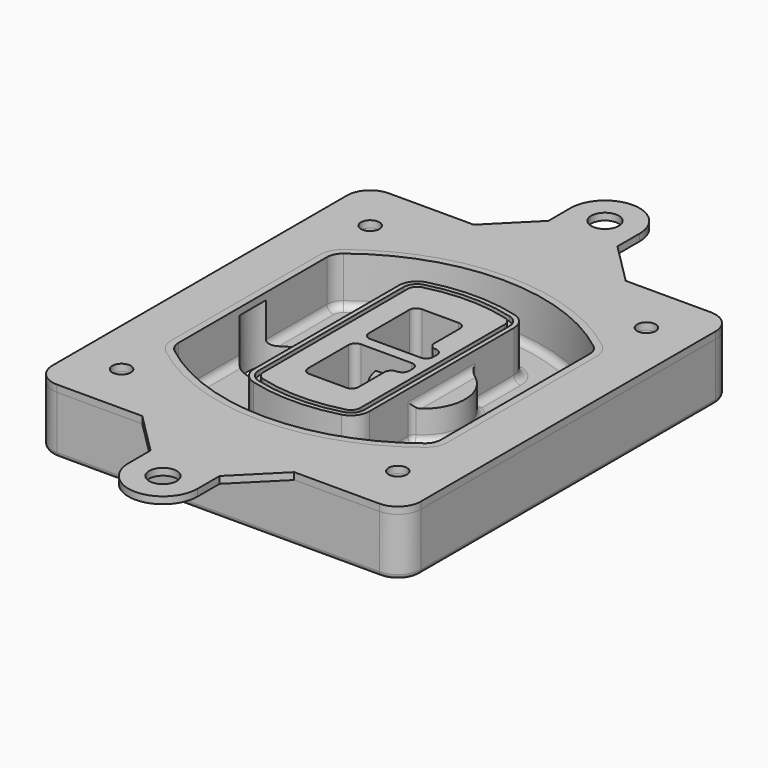
from build123d import *

# Parameters (mm, degrees)
F0_R      = 4
F1_DEPTH  = 25
F2_DEPTH  = 3
F3_DEPTH  = 18
F5_DEPTH  = 21
F6_DEPTH  = 2
F8_DEPTH  = 20
F9_DEPTH  = 16
F10_DEPTH = 25
F7_R      = 6
F7_R_2    = 4
F11_DEPTH = 6
F13_DEPTH = 9
F14_R     = 3
F15_R     = 2
F16_R     = 6
F16_R_2   = 4
F17_DEPTH = 3


with BuildPart() as f1:
    # F0 (on Top) → F1 (new body)
    with BuildSketch(Plane.XY):
        with BuildLine():
            ThreePointArc((-80, -80), (-77.0710678119, -87.0710678119), (-70, -90))
            Line((-70, -90), (70, -90))
            ThreePointArc((70, -90), (77.0710678119, -87.0710678119), (80, -80))
            Line((80, -80), (80, 80))
            ThreePointArc((80, 80), (77.0710678119, 87.0710678119), (70, 90))
            Line((70, 90), (-70, 90))
            ThreePointArc((-70, 90), (-77.0710678119, 87.0710678119), (-80, 80))
            Line((-80, 80), (-80, -80))
        make_face()
        with Locations((-60, -67.5)):
            Circle(F0_R, mode=Mode.SUBTRACT)
        with Locations((60, -67.5)):
            Circle(F0_R, mode=Mode.SUBTRACT)
        with Locations((-60, 67.5)):
            Circle(F0_R, mode=Mode.SUBTRACT)
        with BuildLine():
            ThreePointArc((-64, 40.2934422872), (-62.5820384798, 46.4328484224), (-58.6153846154, 51.3286200352))
            ThreePointArc((-58.6153846154, 51.3286200352), (0, 71.5), (58.6153846154, 51.3286200352))
            ThreePointArc((58.6153846154, 51.3286200352), (62.5820384798, 46.4328484224), (64, 40.2934422872))
            Line((64, 40.2934422872), (64, -40.2934422872))
            ThreePointArc((64, -40.2934422872), (62.5820384798, -46.4328484224), (58.6153846154, -51.3286200352))
            ThreePointArc((58.6153846154, -51.3286200352), (0, -71.5), (-58.6153846154, -51.3286200352))
            ThreePointArc((-58.6153846154, -51.3286200352), (-62.5820384798, -46.4328484224), (-64, -40.2934422872))
            Line((-64, -40.2934422872), (-64, 40.2934422872))
        make_face(mode=Mode.SUBTRACT)
        with Locations((60, 67.5)):
            Circle(F0_R, mode=Mode.SUBTRACT)
        with BuildLine():
            ThreePointArc((58.6153846154, 51.3286200352), (0, 71.5), (-58.6153846154, 51.3286200352))
            ThreePointArc((-58.6153846154, 51.3286200352), (-62.5820384798, 46.4328484224), (-64, 40.2934422872))
            Line((-64, 40.2934422872), (-64, -40.2934422872))
            ThreePointArc((-64, -40.2934422872), (-62.5820384798, -46.4328484224), (-58.6153846154, -51.3286200352))
            ThreePointArc((-58.6153846154, -51.3286200352), (0, -71.5), (58.6153846154, -51.3286200352))
            ThreePointArc((58.6153846154, -51.3286200352), (62.5820384798, -46.4328484224), (64, -40.2934422872))
            Line((64, -40.2934422872), (64, 40.2934422872))
            ThreePointArc((64, 40.2934422872), (62.5820384798, 46.4328484224), (58.6153846154, 51.3286200352))
        make_face()
        with BuildLine():
            Line((-60, -40.2934422872), (-60, 40.2934422872))
            ThreePointArc((-60, 40.2934422872), (-58.9871703427, 44.6787323838), (-56.1538461538, 48.1757121072))
            ThreePointArc((-56.1538461538, 48.1757121072), (0, 67.5), (56.1538461538, 48.1757121072))
            ThreePointArc((56.1538461538, 48.1757121072), (58.9871703427, 44.6787323838), (60, 40.2934422872))
            Line((60, 40.2934422872), (60, -40.2934422872))
            ThreePointArc((60, -40.2934422872), (58.9871703427, -44.6787323838), (56.1538461538, -48.1757121072))
            ThreePointArc((56.1538461538, -48.1757121072), (0, -67.5), (-56.1538461538, -48.1757121072))
            ThreePointArc((-56.1538461538, -48.1757121072), (-58.9871703427, -44.6787323838), (-60, -40.2934422872))
        make_face(mode=Mode.SUBTRACT)
        with BuildLine():
            ThreePointArc((-56.1538461538, 48.1757121072), (-58.9871703427, 44.6787323838), (-60, 40.2934422872))
            Line((-60, 40.2934422872), (-60, -40.2934422872))
            ThreePointArc((-60, -40.2934422872), (-58.9871703427, -44.6787323838), (-56.1538461538, -48.1757121072))
            ThreePointArc((-56.1538461538, -48.1757121072), (0, -67.5), (56.1538461538, -48.1757121072))
            ThreePointArc((56.1538461538, -48.1757121072), (58.9871703427, -44.6787323838), (60, -40.2934422872))
            Line((60, -40.2934422872), (60, 40.2934422872))
            ThreePointArc((60, 40.2934422872), (58.9871703427, 44.6787323838), (56.1538461538, 48.1757121072))
            ThreePointArc((56.1538461538, 48.1757121072), (0, 67.5), (-56.1538461538, 48.1757121072))
        make_face()
        with BuildLine():
            ThreePointArc((54.3076923077, 45.8110311612), (56.2910192399, 43.3631453548), (57, 40.2934422872))
            Line((57, 40.2934422872), (57, -40.2934422872))
            ThreePointArc((57, -40.2934422872), (56.2910192399, -43.3631453548), (54.3076923077, -45.8110311612))
            ThreePointArc((54.3076923077, -45.8110311612), (0, -64.5), (-54.3076923077, -45.8110311612))
            ThreePointArc((-54.3076923077, -45.8110311612), (-56.2910192399, -43.3631453548), (-57, -40.2934422872))
            Line((-57, -40.2934422872), (-57, 40.2934422872))
            ThreePointArc((-57, 40.2934422872), (-56.2910192399, 43.3631453548), (-54.3076923077, 45.8110311612))
            ThreePointArc((-54.3076923077, 45.8110311612), (0, 64.5), (54.3076923077, 45.8110311612))
        make_face(mode=Mode.SUBTRACT)
        with BuildLine():
            Line((57, -40.2934422872), (57, 40.2934422872))
            ThreePointArc((57, 40.2934422872), (56.2910192399, 43.3631453548), (54.3076923077, 45.8110311612))
            ThreePointArc((54.3076923077, 45.8110311612), (0, 64.5), (-54.3076923077, 45.8110311612))
            ThreePointArc((-54.3076923077, 45.8110311612), (-56.2910192399, 43.3631453548), (-57, 40.2934422872))
            Line((-57, 40.2934422872), (-57, -40.2934422872))
            ThreePointArc((-57, -40.2934422872), (-56.2910192399, -43.3631453548), (-54.3076923077, -45.8110311612))
            ThreePointArc((-54.3076923077, -45.8110311612), (0, -64.5), (54.3076923077, -45.8110311612))
            ThreePointArc((54.3076923077, -45.8110311612), (56.2910192399, -43.3631453548), (57, -40.2934422872))
        make_face()
    extrude(amount=-F1_DEPTH)

    # F0 (on Top) → F2 (join)
    with BuildSketch(Plane.XY):
        with BuildLine():
            ThreePointArc((-56.1538461538, 48.1757121072), (-58.9871703427, 44.6787323838), (-60, 40.2934422872))
            Line((-60, 40.2934422872), (-60, -40.2934422872))
            ThreePointArc((-60, -40.2934422872), (-58.9871703427, -44.6787323838), (-56.1538461538, -48.1757121072))
            ThreePointArc((-56.1538461538, -48.1757121072), (0, -67.5), (56.1538461538, -48.1757121072))
            ThreePointArc((56.1538461538, -48.1757121072), (58.9871703427, -44.6787323838), (60, -40.2934422872))
            Line((60, -40.2934422872), (60, 40.2934422872))
            ThreePointArc((60, 40.2934422872), (58.9871703427, 44.6787323838), (56.1538461538, 48.1757121072))
            ThreePointArc((56.1538461538, 48.1757121072), (0, 67.5), (-56.1538461538, 48.1757121072))
        make_face()
        with BuildLine():
            ThreePointArc((54.3076923077, 45.8110311612), (56.2910192399, 43.3631453548), (57, 40.2934422872))
            Line((57, 40.2934422872), (57, -40.2934422872))
            ThreePointArc((57, -40.2934422872), (56.2910192399, -43.3631453548), (54.3076923077, -45.8110311612))
            ThreePointArc((54.3076923077, -45.8110311612), (0, -64.5), (-54.3076923077, -45.8110311612))
            ThreePointArc((-54.3076923077, -45.8110311612), (-56.2910192399, -43.3631453548), (-57, -40.2934422872))
            Line((-57, -40.2934422872), (-57, 40.2934422872))
            ThreePointArc((-57, 40.2934422872), (-56.2910192399, 43.3631453548), (-54.3076923077, 45.8110311612))
            ThreePointArc((-54.3076923077, 45.8110311612), (0, 64.5), (54.3076923077, 45.8110311612))
        make_face(mode=Mode.SUBTRACT)
    extrude(amount=F2_DEPTH)

    # F0 (on Top) → F3 (cut)
    with BuildSketch(Plane.XY):
        with BuildLine():
            Line((57, -40.2934422872), (57, 40.2934422872))
            ThreePointArc((57, 40.2934422872), (56.2910192399, 43.3631453548), (54.3076923077, 45.8110311612))
            ThreePointArc((54.3076923077, 45.8110311612), (0, 64.5), (-54.3076923077, 45.8110311612))
            ThreePointArc((-54.3076923077, 45.8110311612), (-56.2910192399, 43.3631453548), (-57, 40.2934422872))
            Line((-57, 40.2934422872), (-57, -40.2934422872))
            ThreePointArc((-57, -40.2934422872), (-56.2910192399, -43.3631453548), (-54.3076923077, -45.8110311612))
            ThreePointArc((-54.3076923077, -45.8110311612), (0, -64.5), (54.3076923077, -45.8110311612))
            ThreePointArc((54.3076923077, -45.8110311612), (56.2910192399, -43.3631453548), (57, -40.2934422872))
        make_face()
    extrude(amount=-F3_DEPTH, mode=Mode.SUBTRACT)

    # F4 (on face) → F5 (join, through all)
    with BuildSketch(Plane.XY.offset(3)):
        with BuildLine():
            ThreePointArc((-25, -39.2465276821), (-23.3511545998, -44.1109737193), (-19.0842911877, -46.9702398883))
            ThreePointArc((-19.0842911877, -46.9702398883), (0, -49.5), (19.0842911877, -46.9702398883))
            ThreePointArc((19.0842911877, -46.9702398883), (23.3511545998, -44.1109737193), (25, -39.2465276821))
            Line((25, -39.2465276821), (25, 39.2465276821))
            ThreePointArc((25, 39.2465276821), (23.3511545998, 44.1109737193), (19.0842911877, 46.9702398883))
            ThreePointArc((19.0842911877, 46.9702398883), (0, 49.5), (-19.0842911877, 46.9702398883))
            ThreePointArc((-19.0842911877, 46.9702398883), (-23.3511545998, 44.1109737193), (-25, 39.2465276821))
            Line((-25, 39.2465276821), (-25, -39.2465276821))
        make_face()
        with BuildLine():
            ThreePointArc((18.5632183908, 45.0393118368), (21.7633659499, 42.89486221), (23, 39.2465276821))
            Line((23, 39.2465276821), (23, -39.2465276821))
            ThreePointArc((23, -39.2465276821), (21.7633659499, -42.89486221), (18.5632183908, -45.0393118368))
            ThreePointArc((18.5632183908, -45.0393118368), (0, -47.5), (-18.5632183908, -45.0393118368))
            ThreePointArc((-18.5632183908, -45.0393118368), (-21.7633659499, -42.89486221), (-23, -39.2465276821))
            Line((-23, -39.2465276821), (-23, 39.2465276821))
            ThreePointArc((-23, 39.2465276821), (-21.7633659499, 42.89486221), (-18.5632183908, 45.0393118368))
            ThreePointArc((-18.5632183908, 45.0393118368), (0, 47.5), (18.5632183908, 45.0393118368))
        make_face(mode=Mode.SUBTRACT)
        with BuildLine():
            Line((23, -39.2465276821), (23, 39.2465276821))
            ThreePointArc((23, 39.2465276821), (21.7633659499, 42.89486221), (18.5632183908, 45.0393118368))
            ThreePointArc((18.5632183908, 45.0393118368), (0, 47.5), (-18.5632183908, 45.0393118368))
            ThreePointArc((-18.5632183908, 45.0393118368), (-21.7633659499, 42.89486221), (-23, 39.2465276821))
            Line((-23, 39.2465276821), (-23, -39.2465276821))
            ThreePointArc((-23, -39.2465276821), (-21.7633659499, -42.89486221), (-18.5632183908, -45.0393118368))
            ThreePointArc((-18.5632183908, -45.0393118368), (0, -47.5), (18.5632183908, -45.0393118368))
            ThreePointArc((18.5632183908, -45.0393118368), (21.7633659499, -42.89486221), (23, -39.2465276821))
        make_face()
        with BuildLine():
            ThreePointArc((18.0421455939, 43.1083837852), (20.1755772999, 41.6787507007), (21, 39.2465276821))
            Line((21, 39.2465276821), (21, -39.2465276821))
            ThreePointArc((21, -39.2465276821), (20.1755772999, -41.6787507007), (18.0421455939, -43.1083837852))
            ThreePointArc((18.0421455939, -43.1083837852), (0, -45.5), (-18.0421455939, -43.1083837852))
            ThreePointArc((-18.0421455939, -43.1083837852), (-20.1755772999, -41.6787507007), (-21, -39.2465276821))
            Line((-21, -39.2465276821), (-21, 39.2465276821))
            ThreePointArc((-21, 39.2465276821), (-20.1755772999, 41.6787507007), (-18.0421455939, 43.1083837852))
            ThreePointArc((-18.0421455939, 43.1083837852), (0, 45.5), (18.0421455939, 43.1083837852))
        make_face(mode=Mode.SUBTRACT)
        with BuildLine():
            Line((21, -39.2465276821), (21, 39.2465276821))
            ThreePointArc((21, 39.2465276821), (20.1755772999, 41.6787507007), (18.0421455939, 43.1083837852))
            ThreePointArc((18.0421455939, 43.1083837852), (0, 45.5), (-18.0421455939, 43.1083837852))
            ThreePointArc((-18.0421455939, 43.1083837852), (-20.1755772999, 41.6787507007), (-21, 39.2465276821))
            Line((-21, 39.2465276821), (-21, -39.2465276821))
            ThreePointArc((-21, -39.2465276821), (-20.1755772999, -41.6787507007), (-18.0421455939, -43.1083837852))
            ThreePointArc((-18.0421455939, -43.1083837852), (0, -45.5), (18.0421455939, -43.1083837852))
            ThreePointArc((18.0421455939, -43.1083837852), (20.1755772999, -41.6787507007), (21, -39.2465276821))
        make_face()
        with BuildLine():
            Line((-8, -2.5), (14, -2.5))
            ThreePointArc((14, -2.5), (16.1213203436, -3.3786796564), (17, -5.5))
            Line((17, -5.5), (17, -7.5))
            ThreePointArc((17, -7.5), (16.1213203436, -9.6213203436), (14, -10.5))
            ThreePointArc((14, -10.5), (11.8786796564, -11.3786796564), (11, -13.5))
            Line((11, -13.5), (11, -27.5))
            ThreePointArc((11, -27.5), (10.1213203436, -29.6213203436), (8, -30.5))
            Line((8, -30.5), (-8, -30.5))
            ThreePointArc((-8, -30.5), (-10.1213203436, -29.6213203436), (-11, -27.5))
            Line((-11, -27.5), (-11, -5.5))
            ThreePointArc((-11, -5.5), (-10.1213203436, -3.3786796564), (-8, -2.5))
        make_face(mode=Mode.SUBTRACT)
        with BuildLine():
            ThreePointArc((-8, 2.5), (-10.1213203436, 3.3786796564), (-11, 5.5))
            Line((-11, 5.5), (-11, 27.5))
            ThreePointArc((-11, 27.5), (-10.1213203436, 29.6213203436), (-8, 30.5))
            Line((-8, 30.5), (8, 30.5))
            ThreePointArc((8, 30.5), (10.1213203436, 29.6213203436), (11, 27.5))
            Line((11, 27.5), (11, 13.5))
            ThreePointArc((11, 13.5), (11.8786796564, 11.3786796564), (14, 10.5))
            ThreePointArc((14, 10.5), (16.1213203436, 9.6213203436), (17, 7.5))
            Line((17, 7.5), (17, 5.5))
            ThreePointArc((17, 5.5), (16.1213203436, 3.3786796564), (14, 2.5))
            Line((14, 2.5), (-8, 2.5))
        make_face(mode=Mode.SUBTRACT)
    extrude(amount=-F5_DEPTH)

    # F4 (on face) → F6 (cut)
    with BuildSketch(Plane.XY.offset(3)):
        with BuildLine():
            Line((23, -39.2465276821), (23, 39.2465276821))
            ThreePointArc((23, 39.2465276821), (21.7633659499, 42.89486221), (18.5632183908, 45.0393118368))
            ThreePointArc((18.5632183908, 45.0393118368), (0, 47.5), (-18.5632183908, 45.0393118368))
            ThreePointArc((-18.5632183908, 45.0393118368), (-21.7633659499, 42.89486221), (-23, 39.2465276821))
            Line((-23, 39.2465276821), (-23, -39.2465276821))
            ThreePointArc((-23, -39.2465276821), (-21.7633659499, -42.89486221), (-18.5632183908, -45.0393118368))
            ThreePointArc((-18.5632183908, -45.0393118368), (0, -47.5), (18.5632183908, -45.0393118368))
            ThreePointArc((18.5632183908, -45.0393118368), (21.7633659499, -42.89486221), (23, -39.2465276821))
        make_face()
        with BuildLine():
            ThreePointArc((18.0421455939, 43.1083837852), (20.1755772999, 41.6787507007), (21, 39.2465276821))
            Line((21, 39.2465276821), (21, -39.2465276821))
            ThreePointArc((21, -39.2465276821), (20.1755772999, -41.6787507007), (18.0421455939, -43.1083837852))
            ThreePointArc((18.0421455939, -43.1083837852), (0, -45.5), (-18.0421455939, -43.1083837852))
            ThreePointArc((-18.0421455939, -43.1083837852), (-20.1755772999, -41.6787507007), (-21, -39.2465276821))
            Line((-21, -39.2465276821), (-21, 39.2465276821))
            ThreePointArc((-21, 39.2465276821), (-20.1755772999, 41.6787507007), (-18.0421455939, 43.1083837852))
            ThreePointArc((-18.0421455939, 43.1083837852), (0, 45.5), (18.0421455939, 43.1083837852))
        make_face(mode=Mode.SUBTRACT)
    extrude(amount=-F6_DEPTH, mode=Mode.SUBTRACT)

    # F7 (on face) → F8 (join)
    with BuildSketch(Plane(origin=(0, 0, -25), x_dir=(1, 0, 0), z_dir=(0, 0, -1))):
        with BuildLine():
            ThreePointArc((3.28842436, 0), (16.7567035675, 13.4682792075), (30.224982775, 0))
            Line((30.224982775, 0), (35.224982775, 0))
            ThreePointArc((35.224982775, 0), (16.7567035675, 18.4682792075), (-1.71157564, 0))
            Line((-1.71157564, 0), (3.28842436, 0))
        make_face()
        with BuildLine():
            Line((3.28842436, 0), (30.224982775, 0))
            ThreePointArc((30.224982775, 0), (16.7567035675, 13.4682792075), (3.28842436, 0))
        make_face()
        with BuildLine():
            ThreePointArc((3.28842436, 0), (16.7567035675, -13.4682792075), (30.224982775, 0))
            Line((30.224982775, 0), (3.28842436, 0))
        make_face()
        with BuildLine():
            Line((35.224982775, 0), (30.224982775, 0))
            ThreePointArc((30.224982775, 0), (16.7567035675, -13.4682792075), (3.28842436, 0))
            Line((3.28842436, 0), (-1.71157564, 0))
            ThreePointArc((-1.71157564, 0), (16.7567035675, -18.4682792075), (35.224982775, 0))
        make_face()
    extrude(amount=-F8_DEPTH)

    # F7 (on face) → F9 (cut)
    with BuildSketch(Plane(origin=(0, 0, -25), x_dir=(1, 0, 0), z_dir=(0, 0, -1))):
        with BuildLine():
            Line((3.28842436, 0), (30.224982775, 0))
            ThreePointArc((30.224982775, 0), (16.7567035675, 13.4682792075), (3.28842436, 0))
        make_face()
        with BuildLine():
            ThreePointArc((3.28842436, 0), (16.7567035675, -13.4682792075), (30.224982775, 0))
            Line((30.224982775, 0), (3.28842436, 0))
        make_face()
    extrude(amount=-F9_DEPTH, mode=Mode.SUBTRACT)

    # F7 (on face) → F10 (cut)
    with BuildSketch(Plane(origin=(0, 0, -25), x_dir=(1, 0, 0), z_dir=(0, 0, -1))):
        with BuildLine():
            Line((-59.0318229325, 0), (-32.0952645175, 0))
            ThreePointArc((-32.0952645175, 0), (-45.563543725, 13.4682792075), (-59.0318229325, 0))
        make_face()
        with BuildLine():
            ThreePointArc((-59.0318229325, 0), (-45.563543725, -13.4682792075), (-32.0952645175, 0))
            Line((-32.0952645175, 0), (-59.0318229325, 0))
        make_face()
    extrude(amount=-F10_DEPTH, mode=Mode.SUBTRACT)

    # F7 (on face) → F11 (cut)
    with BuildSketch(Plane(origin=(0, 0, -25), x_dir=(1, 0, 0), z_dir=(0, 0, -1))):
        with Locations((60, -67.5)):
            Circle(F7_R)
        with Locations((60, -67.5)):
            Circle(F7_R_2, mode=Mode.SUBTRACT)
        with Locations((-60, -67.5)):
            Circle(F7_R)
        with Locations((-60, -67.5)):
            Circle(F7_R_2, mode=Mode.SUBTRACT)
        with Locations((-60, 67.5)):
            Circle(F7_R)
        with Locations((-60, 67.5)):
            Circle(F7_R_2, mode=Mode.SUBTRACT)
        with Locations((60, 67.5)):
            Circle(F7_R)
        with Locations((60, 67.5)):
            Circle(F7_R_2, mode=Mode.SUBTRACT)
    extrude(amount=-F11_DEPTH, mode=Mode.SUBTRACT)

    # F12 (on face) → F13 (cut, through all)
    with BuildSketch(Plane(origin=(0, 0, -9), x_dir=(1, 0, 0), z_dir=(0, 0, -1))):
        with BuildLine():
            Line((11, 13.5), (11, 17.5481537753))
            ThreePointArc((11, 17.5481537753), (2.5696536419, 11.8239143813), (-1.5415842455, 2.5))
            Line((-1.5415842455, 2.5), (3.5224848595, 2.5))
            ThreePointArc((3.5224848595, 2.5), (6.1857188154, 8.3455872281), (11.2536447004, 12.2927168648))
            ThreePointArc((11.2536447004, 12.2927168648), (11.0640958889, 12.8831798879), (11, 13.5))
        make_face()
        with BuildLine():
            ThreePointArc((11.2536447004, -12.2927168648), (6.1857188154, -8.3455872281), (3.5224848595, -2.5))
            Line((3.5224848595, -2.5), (-1.5415842455, -2.5))
            ThreePointArc((-1.5415842455, -2.5), (2.5696536419, -11.8239143813), (11, -17.5481537753))
            Line((11, -17.5481537753), (11, -13.5))
            ThreePointArc((11, -13.5), (11.0640958889, -12.8831798879), (11.2536447004, -12.2927168648))
        make_face()
        with BuildLine():
            ThreePointArc((11.2536447004, 12.2927168648), (6.1857188154, 8.3455872281), (3.5224848595, 2.5))
            Line((3.5224848595, 2.5), (14, 2.5))
            ThreePointArc((14, 2.5), (16.1213203436, 3.3786796564), (17, 5.5))
            Line((17, 5.5), (17, 7.5))
            ThreePointArc((17, 7.5), (16.1213203436, 9.6213203436), (14, 10.5))
            ThreePointArc((14, 10.5), (12.3601599782, 10.9878446101), (11.2536447004, 12.2927168648))
        make_face()
        with BuildLine():
            Line((14, -2.5), (3.5224848595, -2.5))
            ThreePointArc((3.5224848595, -2.5), (6.1857188154, -8.3455872281), (11.2536447004, -12.2927168648))
            ThreePointArc((11.2536447004, -12.2927168648), (12.3601599782, -10.9878446101), (14, -10.5))
            ThreePointArc((14, -10.5), (16.1213203436, -9.6213203436), (17, -7.5))
            Line((17, -7.5), (17, -5.5))
            ThreePointArc((17, -5.5), (16.1213203436, -3.3786796564), (14, -2.5))
        make_face()
    extrude(amount=F13_DEPTH, mode=Mode.SUBTRACT)

    # F14
    f14_edges = [f1.edges().sort_by_distance(p)[0] for p in [
        (-57, -23.703476, -18),
        (-57, 23.703476, -18),
        (25, 0, -5),
        (25, 16.526506, -11.5),
        (25, -16.526506, -11.5),
        (25, -27.886517, -18),
        (35.224983, 0, -18),
    ]]
    fillet(f14_edges, radius=F14_R)

    # F15
    f15_edges = [f1.edges().sort_by_distance(p)[0] for p in [
        (0, -90, -25),
    ]]
    fillet(f15_edges, radius=F15_R)


with BuildPart() as f17:
    # F16 (on face) → F17 (new body, through all)
    with BuildSketch(Plane.XY):
        with BuildLine():
            ThreePointArc((15, 120), (0, 135), (-15, 120))
            Line((-15, 120), (-15, 108))
            Line((-15, 108), (-33, 90))
            Line((-33, 90), (33, 90))
            Line((33, 90), (15, 108))
            Line((15, 108), (15, 120))
        make_face()
        with Locations((0, 120)):
            Circle(F16_R, mode=Mode.SUBTRACT)
        with BuildLine():
            Line((15, -108), (33, -90))
            Line((33, -90), (-33, -90))
            Line((-33, -90), (-15, -108))
            Line((-15, -108), (-15, -120))
            ThreePointArc((-15, -120), (0, -135), (15, -120))
            Line((15, -120), (15, -108))
        make_face()
        with Locations((0, -120)):
            Circle(F16_R, mode=Mode.SUBTRACT)
        with BuildLine():
            Line((33, 90), (-33, 90))
            Line((-33, 90), (-70, 90))
            ThreePointArc((-70, 90), (-77.0710678119, 87.0710678119), (-80, 80))
            Line((-80, 80), (-80, -80))
            ThreePointArc((-80, -80), (-77.0710678119, -87.0710678119), (-70, -90))
            Line((-70, -90), (-33, -90))
            Line((-33, -90), (33, -90))
            Line((33, -90), (70, -90))
            ThreePointArc((70, -90), (77.0710678119, -87.0710678119), (80, -80))
            Line((80, -80), (80, 80))
            ThreePointArc((80, 80), (77.0710678119, 87.0710678119), (70, 90))
            Line((70, 90), (33, 90))
        make_face()
        with Locations((-60, -67.5)):
            Circle(F16_R_2, mode=Mode.SUBTRACT)
        with Locations((60, -67.5)):
            Circle(F16_R_2, mode=Mode.SUBTRACT)
        with Locations((-60, 67.5)):
            Circle(F16_R_2, mode=Mode.SUBTRACT)
        with BuildLine():
            ThreePointArc((-60, 40.2934422872), (-58.9871703427, 44.6787323838), (-56.1538461538, 48.1757121072))
            ThreePointArc((-56.1538461538, 48.1757121072), (0, 67.5), (56.1538461538, 48.1757121072))
            ThreePointArc((56.1538461538, 48.1757121072), (58.9871703427, 44.6787323838), (60, 40.2934422872))
            Line((60, 40.2934422872), (60, -40.2934422872))
            ThreePointArc((60, -40.2934422872), (58.9871703427, -44.6787323838), (56.1538461538, -48.1757121072))
            ThreePointArc((56.1538461538, -48.1757121072), (0, -67.5), (-56.1538461538, -48.1757121072))
            ThreePointArc((-56.1538461538, -48.1757121072), (-58.9871703427, -44.6787323838), (-60, -40.2934422872))
            Line((-60, -40.2934422872), (-60, 40.2934422872))
        make_face(mode=Mode.SUBTRACT)
        with Locations((60, 67.5)):
            Circle(F16_R_2, mode=Mode.SUBTRACT)
    extrude(amount=F17_DEPTH)


solid = Compound([f1.part, f17.part])
